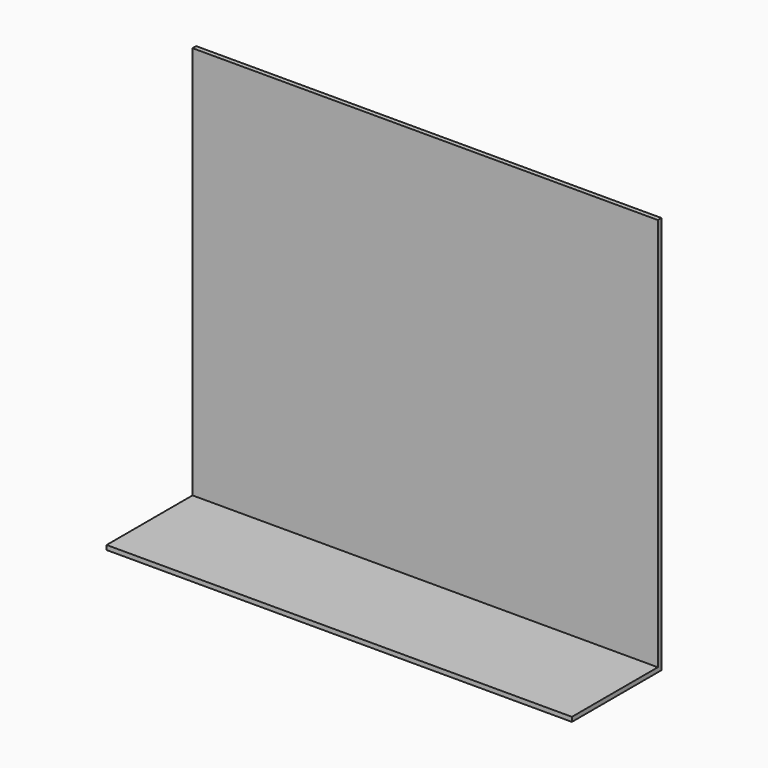
from build123d import *

# Parameters (mm, degrees)
F0_W     = 330.2
F0_H     = 76.2
F1_DEPTH = 3.175
F2_W     = 330.2
F2_H     = 282.575
F3_DEPTH = 3.175


# Not quite as in the source:
# - a length typed as a fraction of an inch, garbled in the dataset ("3 / 203.2 mm" for 3/8 in), is restored


with BuildPart() as f1:
    # F0 (on Top) → F1 (new body)
    with BuildSketch(Plane.XY):
        Rectangle(F0_W, F0_H)
    extrude(amount=F1_DEPTH)

    # F2 (on face) → F3 (join)
    with BuildSketch(Plane(origin=(0, 38.1, 0), x_dir=(-1, 0, 0), z_dir=(0, 1, 0))):
        with Locations((0, 141.2875)):
            Rectangle(F2_W, F2_H)
    extrude(amount=F3_DEPTH)


solid = f1.part
